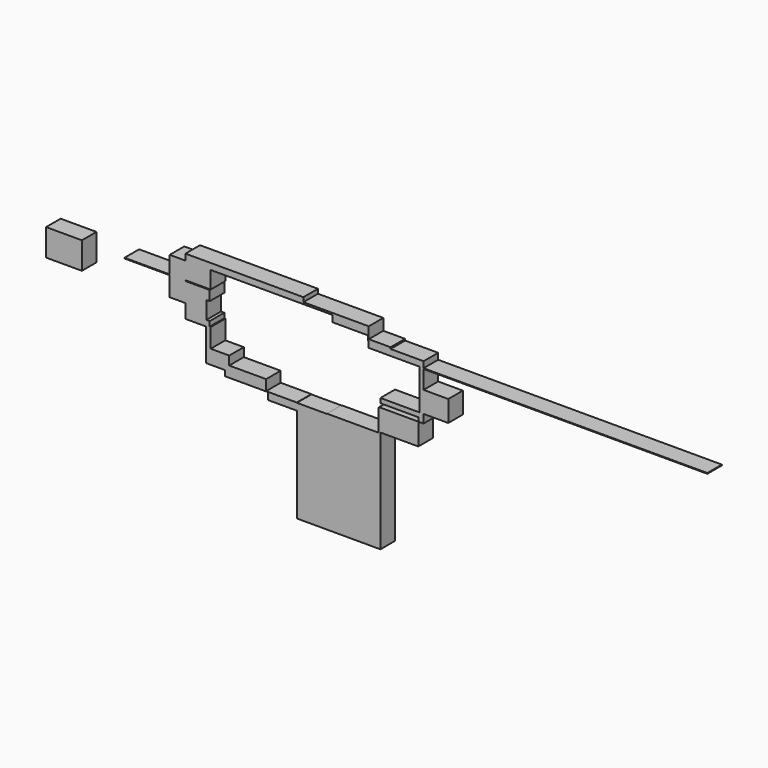
from build123d import *

# Parameters (mm, degrees)
F0_W     = 49.9110035598
F0_H     = 37.4650023878
F1_DEPTH = 25.4
F0_W_2   = 62.9266947508
F0_H_2   = 1.0160021484
F0_W_3   = 21.9223797321
F0_H_3   = 24.016302079
F0_W_4   = 35.2101027966
F0_H_4   = 27.0532034338
F0_W_5   = 0.7122159004
F0_H_5   = 2.1552592516
F0_W_6   = 30.3827822208
F0_H_6   = 8.570253849
F0_W_7   = 40.5665338039
F0_W_8   = 40.4263734818
F0_H_7   = 0.3592148423
F0_H_8   = 9.6986740828
F0_W_9   = 5.4933428764
F0_W_10  = 395.4214453697
F0_H_9   = 25.6163654849
F0_H_10  = 29.4552231207
F0_W_11  = 34.3640446663
F0_H_11  = 11.8539407849
F0_W_12  = 52.7721643448
F0_H_12  = 30.1736667752
F0_W_13  = 1.9087791443
F0_H_13  = 0.3592073917


# Not quite as in the source:
# - ends of sketch curves that miss each other by under 0.0002 mm in the source are joined


with BuildPart() as f1:
    # F0 (on Front) → F1 (new body)
    with BuildSketch(Plane.XZ):
        with Locations((24.9555017799, 18.7325011939)):
            Rectangle(F0_W, F0_H)
    extrude(amount=F1_DEPTH)


with BuildPart() as f1b:
    # F0 (on Front) → F1, piece 2 (new body)
    with BuildSketch(Plane.XZ):
        with Locations((140.8103480935, 34.9250007421)):
            Rectangle(F0_W_2, F0_H_2)
        with Locations((183.234885335, 47.4411528558)):
            Rectangle(F0_W_3, F0_H_3)
        with Locations((183.234885335, 34.9250007421)):
            Rectangle(F0_W_3, F0_H_2)
        with Locations((211.8011265993, 47.4411528558)):
            Rectangle(F0_W_4, F0_H_3)
        with Locations((183.234885335, 20.890397951)):
            Rectangle(F0_W_3, F0_H_4)
        Polygon((227.9811799526, 34.4169996679), (194.196075201, 34.4169996679), (194.196075201, 7.3637962341), (223.4135717154, 7.3637962341), (223.4135717154, 20.6545889378), (227.9811799526, 20.6545889378), align=None)
        Polygon((194.196075201, 68.0703520775), (194.196075201, 59.4493038952), (229.4061779976, 59.4493038952), (229.4061779976, 61.9637668133), (358.6011528969, 61.9637668133), (358.6011528969, 68.0703520775), align=None)
        Polygon((229.4061779976, 61.9637668133), (229.4061779976, 59.4493038952), (231.9025844336, 59.4493038952), (358.6011528969, 59.4493038952), (358.6011528969, 61.9637668133), align=None)
        Polygon((223.4135717154, 7.3637962341), (194.196075201, 7.3637962341), (194.196075201, -12.0335444808), (222.7686345577, -12.0335444808), (222.7686345577, -4.849344492), (227.9811799526, -4.849344492), (227.9811799526, -3.7717141677), (223.4135717154, -3.7717141677), align=None)
        Polygon((358.6011528969, 61.9637668133), (358.6011528969, 59.4493001699), (377.9325187206, 59.4493038952), (398.8327085972, 59.4492964447), (398.8327085972, 50.4690408707), (448.9478468895, 50.4690408707), (448.9478468895, 46.1585149169), (449.6600627899, 46.1585149169), (449.6600627899, 61.9637668133), align=None)
        Polygon((229.4061779976, -12.0335444808), (222.7686345577, -12.0335444808), (222.7686345577, -56.9348335266), (249.0781396627, -56.9348335266), (249.0781396627, -37.1782630682), (229.4061779976, -37.1782630682), align=None)
        Polygon((222.7686345577, -4.849344492), (222.7686345577, -12.0335444808), (229.4061779976, -12.0335444808), (229.4061779976, -10.5967074633), (227.9811799526, -10.5967074633), (227.9811799526, -4.849344492), align=None)
        with Locations((449.3039548397, 45.0808852911)):
            Rectangle(F0_W_5, F0_H_5)
        with Locations((464.8514539003, 45.0808852911)):
            Rectangle(F0_W_6, F0_H_5)
        Polygon((249.0781396627, -37.1782630682), (249.0781396627, -56.9348335266), (306.6283762455, -56.9348335266), (306.6283762455, -49.3914186954), (255.2164494991, -49.3914186954), (255.2164494991, -37.1782630682), align=None)
        Polygon((306.6283762455, -56.9348335266), (249.0781396627, -56.9348335266), (249.0781396627, -64.4782409072), (308.9790642262, -64.4782409072), (308.9790642262, -64.1190260649), (306.6283762455, -64.1190260649), align=None)
        with Locations((464.8514539003, 39.7181287408)):
            Rectangle(F0_W_6, F0_H_6)
        with Locations((500.3261119127, 39.7181287408)):
            Rectangle(F0_W_7, F0_H_6)
        with Locations((329.192250967, -64.298633486)):
            Rectangle(F0_W_8, F0_H_7)
        with Locations((329.192250967, -69.3275779486)):
            Rectangle(F0_W_8, F0_H_8)
        with Locations((523.3560502529, 39.7181287408)):
            Rectangle(F0_W_9, F0_H_6)
        Polygon((391.3746476173, -64.4782409072), (349.4054377079, -64.4782409072), (349.4054377079, -74.1769149899), (443.1339204311, -74.1769149899), (443.1339204311, -64.1190260649), (391.3746476173, -64.1190260649), align=None)
        with Locations((523.3560502529, 34.9250007421)):
            Rectangle(F0_W_9, F0_H_2)
        Polygon((443.1339204311, -74.1769149899), (349.4054377079, -74.1769149899), (349.4054377079, -206.3867151737), (465.9284353256, -206.3867151737), (465.9284353256, -63.0414038897), (462.9626870155, -63.0414038897), (462.9626870155, -64.1190260649), (443.1339204311, -64.1190260649), align=None)
        with Locations((723.813444376, 34.9250007421)):
            Rectangle(F0_W_10, F0_H_2)
        with Locations((523.3560502529, 21.6088169254)):
            Rectangle(F0_W_9, F0_H_9)
        with Locations((523.3560502529, -5.9269773774)):
            Rectangle(F0_W_9, F0_H_10)
        with Locations((543.2847440243, -5.9269773774)):
            Rectangle(F0_W_11, F0_H_10)
        with Locations((523.3560502529, -26.5815593302)):
            Rectangle(F0_W_9, F0_H_11)
        Polygon((520.6093788147, -32.5085297227), (520.6093788147, -20.6545889378), (465.9284353256, -20.6545889378), (465.9284353256, -27.1203722805), (518.7005996704, -27.1203722805), (518.7005996704, -32.5085297227), align=None)
        with Locations((492.314517498, -47.954570502)):
            Rectangle(F0_W_12, F0_H_12)
        Polygon((462.9626870155, -63.0414038897), (465.9284353256, -63.0414038897), (465.9284353256, -32.8677371144), (463.5714888573, -32.8677371144), (463.5714888573, -43.6440333724), (462.9626870155, -43.6440333724), align=None)
        with Locations((519.6549892426, -32.6881334186)):
            Rectangle(F0_W_13, F0_H_13)
        with Locations((492.314517498, -32.6881334186)):
            Rectangle(F0_W_12, F0_H_13)
    extrude(amount=F1_DEPTH)


solid = Compound([f1.part, f1b.part])
